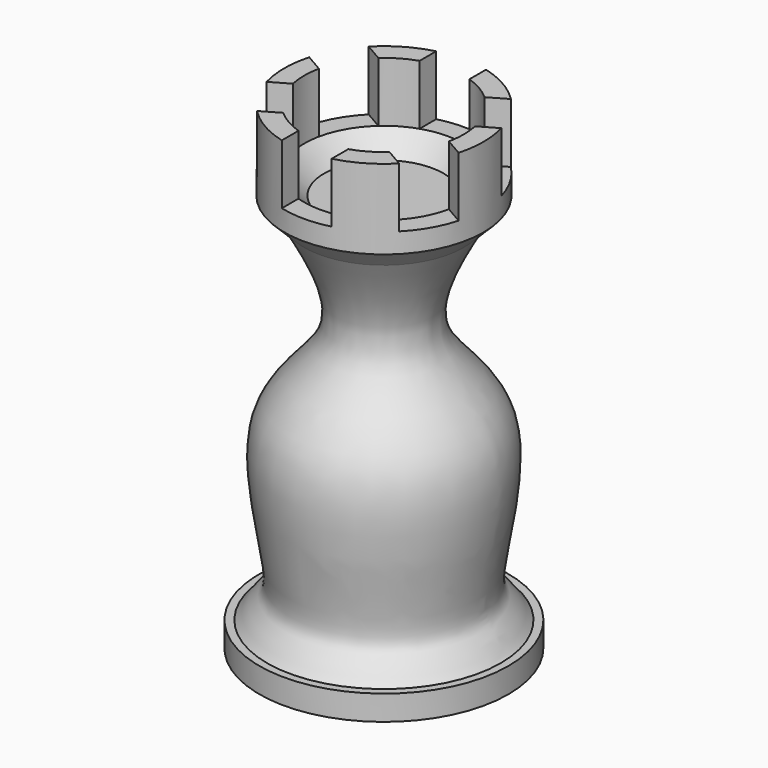
from build123d import *

# Parameters (mm, degrees)
F2_W            = 5
F2_H            = 30
F3_DEPTH        = 6
F3_COPIES_COUNT = 3
F3_COPIES_ANGLE = 120
F4_SIZE         = 1.99999


# Not quite as in the source:
# - a fillet or chamfer is up to 0.001 mm smaller than in the source, because OpenCascade refuses the exact size
# - a pattern or mirror of a feature is missing from the dataset's text; its kind, count and spacing are read off the source's solid


with BuildPart() as f1:
    # F0 (on Front) → F1 (revolve)
    with BuildSketch(Plane.XZ):
        Polygon((0, 40), (0, 38), (8, 38), (10, 40), (10, 48), (8, 48), (8, 40), align=None)
        with BuildLine():
            Line((0, 38), (0, 2.5))
            Line((0, 2.5), (11.7253540084, 2.5))
            add(Edge.make_bspline(
                [(8, 38), (6.2228254188, 34.8766301545), (2.1938698076, 27.4287310591), (13.6516672404, 21.568683637), (8.2315945595, 5.4062057468), (10.5238930021, 4.3384396227), (11.3836559881, 2.7117140323), (11.7253540084, 2.5)],
                knots=[0, 0, 0, 0, 0.246007455, 0.4901278409, 0.783102311, 0.8910484418, 1, 1, 1, 1], degree=3))
            Line((8, 38), (0, 38))
        make_face()
        Polygon((0, 2.5), (0, 0), (12.5, 0), (12.5, 2.5), (11.7253540084, 2.5), align=None)
    revolve(axis=Axis((0, 0, 44), (0, 0, -1)))

    # F2 (on face) → F3 (cut)
    with BuildSketch(Plane.XY.offset(48)):
        Rectangle(F2_W, F2_H)
    f3 = extrude(amount=-F3_DEPTH, mode=Mode.SUBTRACT)

    # F3_copies: F3 ×3 about axis
    f3_copies_axis = Axis((0, 0, 0), (0, 0, 1))
    for i in range(1, F3_COPIES_COUNT):
        add(f3.rotate(f3_copies_axis, i * F3_COPIES_ANGLE / (F3_COPIES_COUNT - 1)), mode=Mode.SUBTRACT)

    # F4 (size 2 in the source; OpenCascade refuses exactly that, so slightly less here)
    f4_edges = [f1.edges().sort_by_distance(p)[0] for p in [
        (-8, 0, 40),
    ]]
    chamfer(f4_edges, length=F4_SIZE)


solid = f1.part
